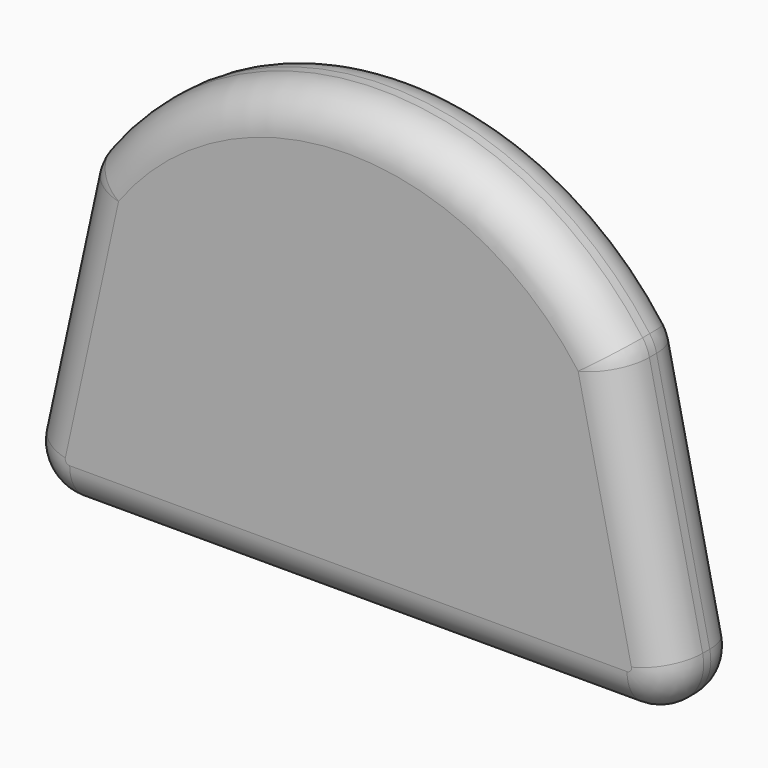
from build123d import *

# Parameters (mm, degrees)
F1_DEPTH = 20
F2_F1_R  = 9
F2_F2_R  = 9
F2_F3_R  = 9
F2_F4_R  = 9
F4_DEPTH = 50


# Not quite as in the source:
# - a feature names something its author has since deleted; it is built from what else it names


with BuildPart() as f1:
    # F0 (on Front) → F1 (new body)
    with BuildSketch(Plane.XZ):
        with BuildLine():
            ThreePointArc((2.6565660371, 12.138023602), (4.6349491554, 3.7302406753), (12.4253354109, 0))
            Line((12.4253354109, 0), (137.5746645891, 0))
            ThreePointArc((137.5746645891, 0), (145.3650508446, 3.7302406753), (147.3434339629, 12.138023602))
            Line((147.3434339629, 12.138023602), (135, 68.5359789614))
            ThreePointArc((135, 68.5359789614), (75, 100), (15, 68.5359789614))
            Line((15, 68.5359789614), (2.6565660371, 12.138023602))
        make_face()
    extrude(amount=F1_DEPTH)

    # F2: fillet of radius 9 on 13 edges, made by hand

    # F2_f1
    f2_f1_edges = [f1.edges().sort_by_distance(p)[0] for p in [
        (135, -10, 68.5359789614),
    ]]
    fillet(f2_f1_edges, radius=F2_F1_R)

    # F2_f2
    f2_f2_edges = [f1.edges().sort_by_distance(p)[0] for p in [
        (15, -10, 68.5359789614),
    ]]
    fillet(f2_f2_edges, radius=F2_F2_R)

    # F2_f3
    f2_f3_edges = [f1.edges().sort_by_distance(p)[0] for p in [
        (75, 0, 100),
    ]]
    fillet(f2_f3_edges, radius=F2_F3_R)

    # F2_f4
    f2_f4_edges = [f1.edges().sort_by_distance(p)[0] for p in [
        (75, -20, 100),
    ]]
    fillet(f2_f4_edges, radius=F2_F4_R)

    # F3 (on face) → F4 (cut)
    with BuildSketch(Plane(origin=(0, 0, 0), x_dir=(1, 0, 0), z_dir=(0, 0, -1))):
        with BuildLine():
            Line((29.25, 5.75), (120.75, 5.75))
            ThreePointArc((120.75, 5.75), (125, 10), (120.75, 14.25))
            Line((120.75, 14.25), (29.25, 14.25))
            ThreePointArc((29.25, 14.25), (25, 10), (29.25, 5.75))
        make_face()
    extrude(amount=-F4_DEPTH, mode=Mode.SUBTRACT)


solid = f1.part
